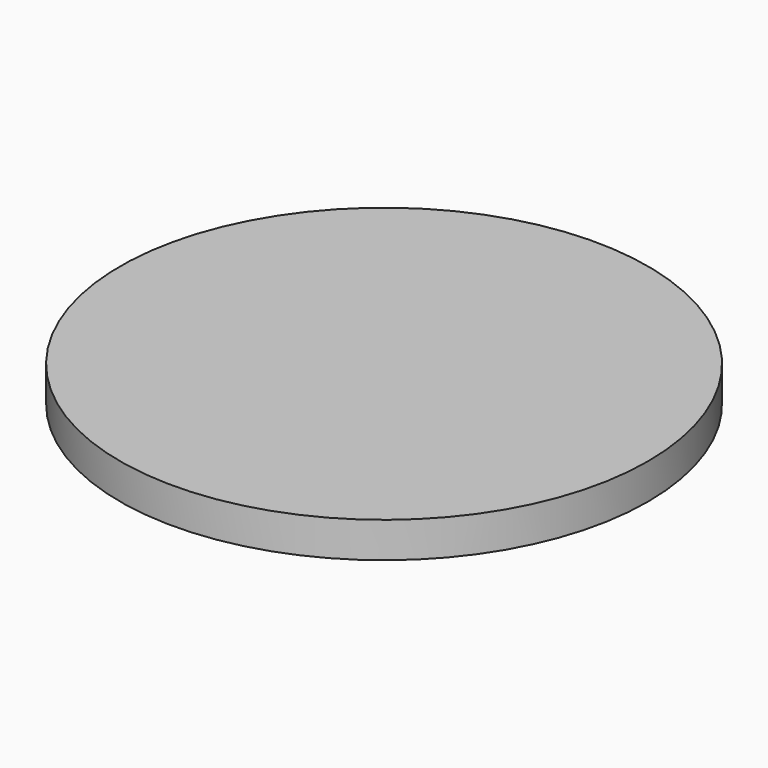
from build123d import *

# Parameters (mm, degrees)
F0_R     = 148.5
F1_DEPTH = 20
F2_R     = 146.5
F2_R_2   = 142
F3_DEPTH = 5


# Not quite as in the source:
# - a feature names something its author has since deleted; it is built from what else it names


with BuildPart() as f1:
    # F0 (on Top) → F1 (new body)
    with BuildSketch(Plane.XY):
        Circle(F0_R)
    extrude(amount=F1_DEPTH)

    # F2 (on face) → F3 (cut)
    with BuildSketch(Plane.XY):
        Circle(F2_R)
        Circle(F2_R_2, mode=Mode.SUBTRACT)
    extrude(amount=F3_DEPTH, mode=Mode.SUBTRACT)


solid = f1.part
